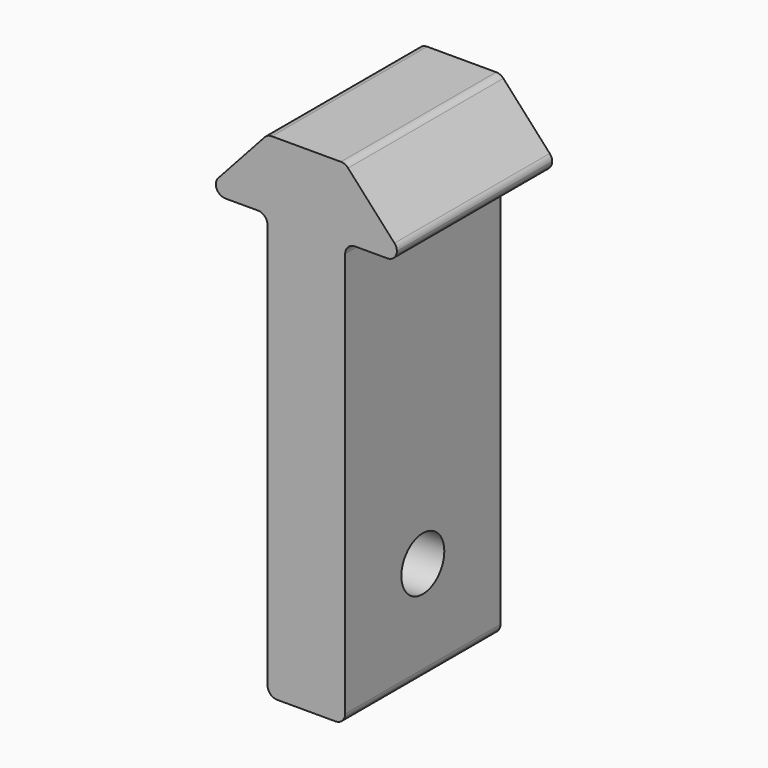
from build123d import *

# Parameters (mm, degrees)
F0_W        = 6
F0_H        = 20.5
F0_H_2      = 4
F0_H_3      = 6
F1_DEPTH    = 15
F2_T1_DEPTH = 15
F2_T3_DEPTH = 16.4497757802
F2_T5_DEPTH = 16.6588870729
F2_T7_DEPTH = 18.75
F3_R        = 2.075
F4_DEPTH    = 12.5


# Not quite as in the source:
# - a fillet or chamfer that OpenCascade refuses, or shapes differently, is made with other operations: its cross-section is extruded or revolved along the edge and cut away or added


with BuildPart() as f1:
    # F0 (on Front) → F1 (new body)
    with BuildSketch(Plane.XZ):
        Polygon((-3, 2.3), (-3, 0), (3, 0), (3, 2.3), (7, 2.3), (7, 3.3), (3, 7.7), (-3, 7.7), (-7, 3.3), (-7, 2.3), align=None)
        with Locations((0, -10.25)):
            Rectangle(F0_W, F0_H)
        with Locations((0, -22.5)):
            Rectangle(F0_W, F0_H_2)
        with Locations((0, -27.5)):
            Rectangle(F0_W, F0_H_3)
    extrude(amount=F1_DEPTH)

    # F2: fillet of radius 0.75 on 10 edges, made by hand

    # F2_s2 → F2_t1 (join)
    with BuildSketch(Plane.XZ):
        with BuildLine():
            ThreePointArc((-3, 1.55), (-3.2196699141, 2.0803300859), (-3.75, 2.3))
            Line((-3.75, 2.3), (-3, 2.3))
            Line((-3, 2.3), (-3, 1.55))
        make_face()
        with BuildLine():
            ThreePointArc((3, 1.55), (3.2196699141, 2.0803300859), (3.75, 2.3))
            Line((3.75, 2.3), (3, 2.3))
            Line((3, 2.3), (3, 1.55))
        make_face()
    extrude(amount=F2_T1_DEPTH)

    # F2_s4 → F2_t3 (cut)
    with BuildSketch(Plane.XZ.offset(-0.7248878901)):
        with BuildLine():
            ThreePointArc((7, 3.010044844), (6.9495413824, 3.2804923515), (6.804955055, 3.5145494394))
            Line((6.804955055, 3.5145494394), (7, 3.3))
            Line((7, 3.3), (7, 3.010044844))
        make_face()
        with BuildLine():
            ThreePointArc((-6.804955055, 3.5145494394), (-6.9495413824, 3.2804923515), (-7, 3.010044844))
            Line((-7, 3.010044844), (-7, 3.3))
            Line((-7, 3.3), (-6.804955055, 3.5145494394))
        make_face()
    extrude(amount=F2_T3_DEPTH, mode=Mode.SUBTRACT)

    # F2_s6 → F2_t5 (cut)
    with BuildSketch(Plane.XZ.offset(-0.8294435365)):
        with BuildLine():
            ThreePointArc((3.2231776405, 7.4545045955), (2.971637774, 7.6358857218), (2.6682225854, 7.7))
            Line((2.6682225854, 7.7), (3, 7.7))
            Line((3, 7.7), (3.2231776405, 7.4545045955))
        make_face()
        with BuildLine():
            ThreePointArc((-2.6682225854, 7.7), (-2.971637774, 7.6358857218), (-3.2231776405, 7.4545045955))
            Line((-3.2231776405, 7.4545045955), (-3, 7.7))
            Line((-3, 7.7), (-2.6682225854, 7.7))
        make_face()
    extrude(amount=F2_T5_DEPTH, mode=Mode.SUBTRACT)

    # F2_s8 → F2_t7 (cut)
    with BuildSketch(Plane.XZ.offset(-1.875)):
        with BuildLine():
            ThreePointArc((-7, 3.05), (-6.7803300859, 2.5196699141), (-6.25, 2.3))
            Line((-6.25, 2.3), (-7, 2.3))
            Line((-7, 2.3), (-7, 3.05))
        make_face()
        with BuildLine():
            ThreePointArc((6.25, 2.3), (6.7803300859, 2.5196699141), (7, 3.05))
            Line((7, 3.05), (7, 2.3))
            Line((7, 2.3), (6.25, 2.3))
        make_face()
        with BuildLine():
            ThreePointArc((2.25, -30.5), (2.7803300859, -30.2803300859), (3, -29.75))
            Line((3, -29.75), (3, -30.5))
            Line((3, -30.5), (2.25, -30.5))
        make_face()
        with BuildLine():
            ThreePointArc((-3, -29.75), (-2.7803300859, -30.2803300859), (-2.25, -30.5))
            Line((-2.25, -30.5), (-3, -30.5))
            Line((-3, -30.5), (-3, -29.75))
        make_face()
    extrude(amount=F2_T7_DEPTH, mode=Mode.SUBTRACT)

    # F3 (on Right) → F4 (cut, symmetric)
    with BuildSketch(Plane.YZ):
        with Locations((-7.5, -22.575)):
            Circle(F3_R)
    extrude(amount=F4_DEPTH, both=True, mode=Mode.SUBTRACT)


solid = f1.part
